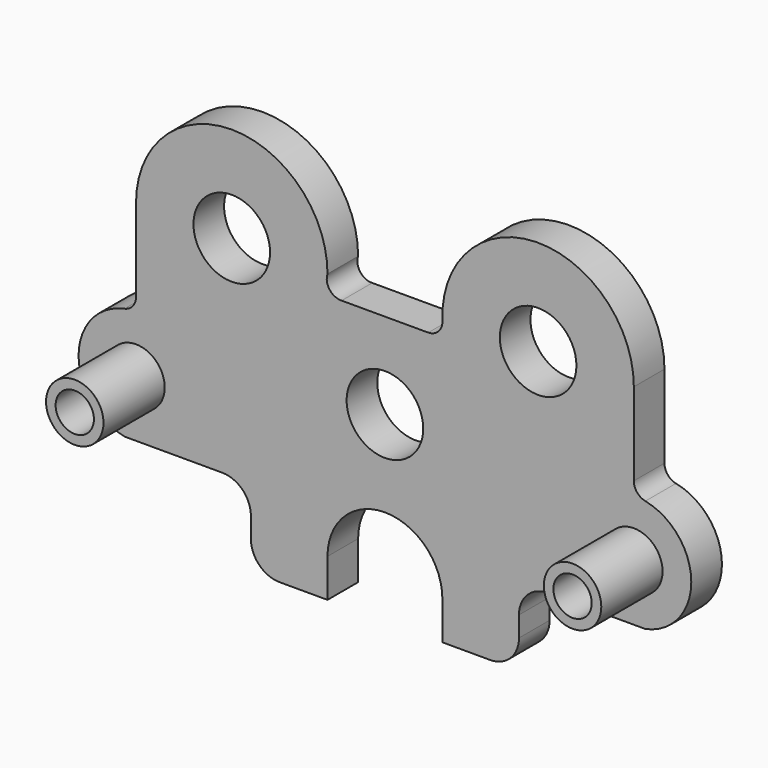
from build123d import *

# Parameters (mm, degrees)
F0_R     = 9.525
F0_R_2   = 12.7
F1_DEPTH = 12.7
F0_R_3   = 6.35
F2_DEPTH = 38.1


with BuildPart() as f1:
    # F0 (on Front) → F1 (new body)
    with BuildSketch(Plane.XZ):
        with BuildLine():
            ThreePointArc((19.0800315969, 33.5443825636), (17.7775003101, 30.0599167658), (14.3667655142, 28.575))
            Line((14.3667655142, 28.575), (-14.3667655142, 28.575))
            ThreePointArc((-14.3667655142, 28.575), (-18.3550358696, 30.4875726696), (-19.0500754755, 34.8557707639))
            ThreePointArc((-19.0500754755, 34.8557707639), (-50.7653853614, 66.6749811311), (-82.55, 34.925))
            Line((-82.55, 34.925), (-82.55, 7.4563898))
            ThreePointArc((-82.55, 7.4563898), (-83.6234833627, 4.4443203287), (-86.36, 2.79011184))
            ThreePointArc((-86.36, 2.79011184), (-101.6, -15.875), (-86.36, -34.54011184))
            Line((-86.36, -34.54011184), (-53.975, -34.54011184))
            ThreePointArc((-53.975, -34.54011184), (-47.2398079092, -37.3299197492), (-44.45, -44.06511184))
            Line((-44.45, -44.06511184), (-44.45, -50.8))
            ThreePointArc((-44.45, -50.8), (-41.6601920908, -57.5351920908), (-34.925, -60.325))
            Line((-34.925, -60.325), (-19.05, -60.325))
            Line((-19.05, -60.325), (-19.05, -47.625))
            ThreePointArc((-19.05, -47.625), (-13.4703841816, -34.1546158184), (0, -28.575))
            ThreePointArc((0, -28.575), (13.4703841816, -34.1546158184), (19.05, -47.625))
            Line((19.05, -47.625), (19.05, -60.325))
            Line((19.05, -60.325), (34.925, -60.325))
            ThreePointArc((34.925, -60.325), (41.6601920908, -57.5351920908), (44.45, -50.8))
            Line((44.45, -50.8), (44.45, -44.06511184))
            ThreePointArc((44.45, -44.06511184), (47.2398079092, -37.3299197492), (53.975, -34.54011184))
            Line((53.975, -34.54011184), (86.36, -34.54011184))
            ThreePointArc((86.36, -34.54011184), (101.6, -15.875), (86.36, 2.79011184))
            ThreePointArc((86.36, 2.79011184), (83.6234833627, 4.4443203287), (82.55, 7.4563898))
            Line((82.55, 7.4563898), (82.55, 34.925))
            ThreePointArc((82.55, 34.925), (50.1095279871, 66.6674912129), (19.0800315969, 33.5443825636))
        make_face()
        with Locations((-82.55, -15.875)):
            Circle(F0_R, mode=Mode.SUBTRACT)
        Circle(F0_R_2, mode=Mode.SUBTRACT)
        with Locations((82.55, -15.875)):
            Circle(F0_R, mode=Mode.SUBTRACT)
        with Locations((-50.8, 34.925)):
            Circle(F0_R_2, mode=Mode.SUBTRACT)
        with Locations((50.8, 34.925)):
            Circle(F0_R_2, mode=Mode.SUBTRACT)
    extrude(amount=F1_DEPTH)

    # F0 (on Front) → F2 (join)
    with BuildSketch(Plane.XZ):
        with Locations((-82.55, -15.875)):
            Circle(F0_R)
        with Locations((-82.55, -15.875)):
            Circle(F0_R_3, mode=Mode.SUBTRACT)
        with Locations((82.55, -15.875)):
            Circle(F0_R)
        with Locations((82.55, -15.875)):
            Circle(F0_R_3, mode=Mode.SUBTRACT)
    extrude(amount=F2_DEPTH)


solid = f1.part
